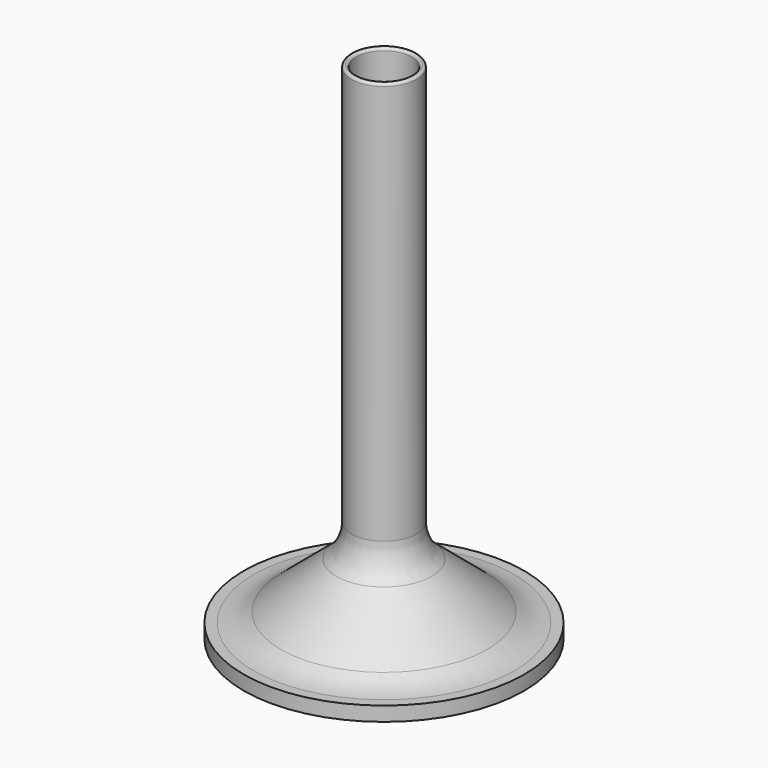
from build123d import *

# Parameters (mm, degrees)
F2_T     = -1.2
F3_R     = 33.2
F3_R_2   = 24.5
F4_DEPTH = 3
F5_R     = 0.59999
F6_R     = 10


# Not quite as in the source:
# - a fillet or chamfer is up to 0.001 mm smaller than in the source, because OpenCascade refuses the exact size


with BuildPart() as f1:
    # F0 (on Front) → F1 (revolve)
    with BuildSketch(Plane.XZ):
        Polygon((-33.2, 0), (0, 0), (0, 119.7204878264), (-7.75, 119.7204878264), (-7.75, 19.7204878264), (-27.2, 3.4), (-33.2, 3.4), align=None)
    revolve(axis=Axis((0, 0, 59.8602439132), (0, 0, -1)))

    # F2
    f2_openings = [f1.faces().sort_by_distance(p)[0] for p in [
        (0, 0, 0),
        (0, 0, 119.720488),
    ]]
    offset(amount=F2_T, openings=f2_openings, kind=Kind.INTERSECTION)

    # F3 (on Top) → F4 (join)
    with BuildSketch(Plane.XY):
        Circle(F3_R)
        Circle(F3_R_2, mode=Mode.SUBTRACT)
    extrude(amount=F4_DEPTH)

    # F5 (radius 0.6 in the source; OpenCascade refuses exactly that, so slightly less here)
    f5_edges = [f1.edges().sort_by_distance(p)[0] for p in [
        (6.55, 0, 119.720488),
        (7.75, 0, 119.720488),
    ]]
    fillet(f5_edges, radius=F5_R)

    # F6
    f6_edges = [f1.edges().sort_by_distance(p)[0] for p in [
        (7.75, 0, 19.720488),
        (27.2, 0, 3.4),
        (-17.475, 0, 11.560244),
    ]]
    fillet(f6_edges, radius=F6_R)


solid = f1.part
